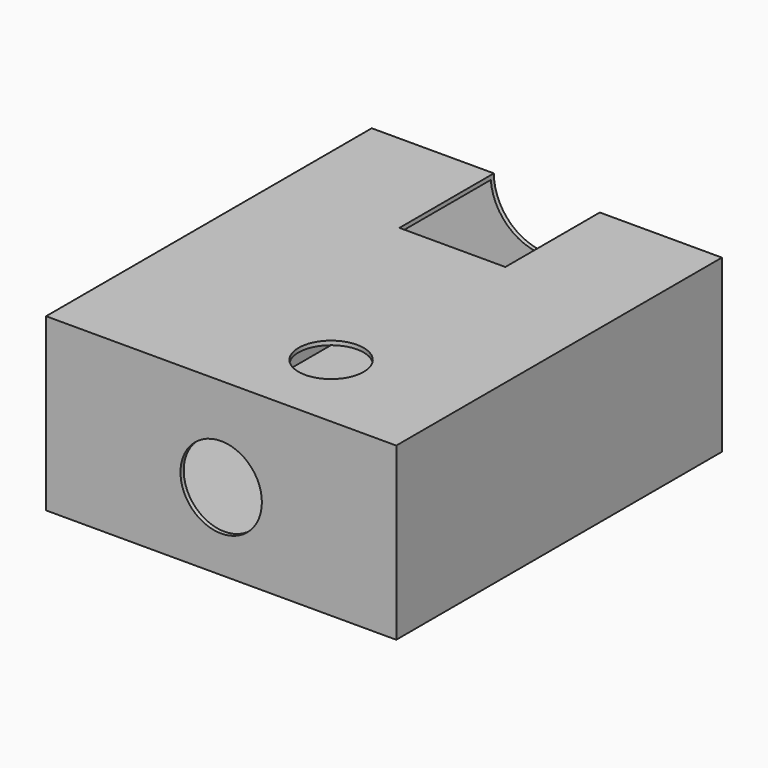
from build123d import *

# Parameters (mm, degrees)
F1_DEPTH = 500
F2_T     = -5
F4_DEPTH = 5
F5_DEPTH = 10
F6_W     = 130.1
F6_H     = 350
F7_DEPTH = 5
F8_R     = 40
F9_DEPTH = 25


# Not quite as in the source:
# - a feature names something its author has since deleted; it is built from what else it names


with BuildPart() as f1:
    # F0 (on Front) → F1 (new body)
    with BuildSketch(Plane.XZ):
        with BuildLine():
            Line((-133.7995099491, 37.318477902), (-133.7995099491, -172.681522098))
            Line((-133.7995099491, -172.681522098), (296.3004900509, -172.681522098))
            Line((296.3004900509, -172.681522098), (296.3004900509, 37.318477902))
            Line((296.3004900509, 37.318477902), (146.3004900509, 37.318477902))
            ThreePointArc((146.3004900509, 37.318477902), (81.2504900509, -27.731522098), (16.2004900509, 37.318477902))
            Line((16.2004900509, 37.318477902), (-133.7995099491, 37.318477902))
        make_face()
    extrude(amount=F1_DEPTH)

    # F2
    f2_openings = [f1.faces().sort_by_distance(p)[0] for p in [
        (81.25049, -250, -27.731522),
    ]]
    offset(amount=F2_T, openings=f2_openings)

    # F3 (on face) → F4 (join)
    with BuildSketch(Plane.XZ.offset(500)):
        with BuildLine():
            Line((146.3004900509, 37.318477902), (16.2004900509, 37.318477902))
            ThreePointArc((16.2004900509, 37.318477902), (35.2531939347, -8.6788182142), (81.2504900509, -27.731522098))
            ThreePointArc((81.2504900509, -27.731522098), (127.2477861671, -8.6788182142), (146.3004900509, 37.318477902))
        make_face()
    extrude(amount=-F4_DEPTH)

    # F3 (on face) → F5 (cut)
    with BuildSketch(Plane.XZ.offset(500)):
        with BuildLine():
            ThreePointArc((81.2504900509, -27.731522098), (45.8951509916, -113.0868611574), (131.2504900509, -77.731522098))
            ThreePointArc((131.2504900509, -77.731522098), (116.6058291102, -42.3761830387), (81.2504900509, -27.731522098))
        make_face()
    extrude(amount=-F5_DEPTH, mode=Mode.SUBTRACT)

    # F6 (on face) → F7 (join)
    with BuildSketch(Plane.XY.offset(37.318477902)):
        with Locations((81.2504900509, -320)):
            Rectangle(F6_W, F6_H)
    extrude(amount=-F7_DEPTH)

    # F8 (on face) → F9 (cut)
    with BuildSketch(Plane.XY.offset(37.318477902)):
        with Locations((136.3004900509, -400)):
            Circle(F8_R)
    extrude(amount=-F9_DEPTH, mode=Mode.SUBTRACT)


solid = f1.part
